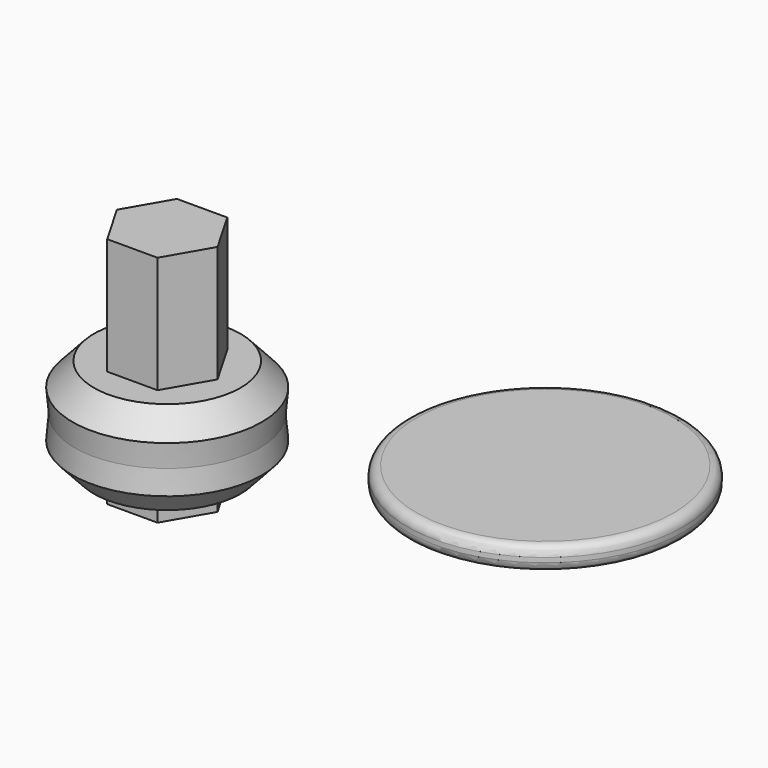
from build123d import *

# Parameters (mm, degrees)
F0_R     = 50.3856473316
F1_DEPTH = 25.4
F1_TAPER = -5
F0_R_2   = 75.1170486434
F2_DEPTH = 6.35
F4_DEPTH = 63.5
F6_R     = 5.08


# Not quite as in the source:
# - a fillet or chamfer that OpenCascade refuses, or shapes differently, is made with other operations: its cross-section is extruded or revolved along the edge and cut away or added


with BuildPart() as f1:
    # F0 (on Top) → F1 (new body, symmetric)
    with BuildSketch(Plane.XY):
        Circle(F0_R)
    extrude(amount=F1_DEPTH, both=True, taper=F1_TAPER)

    # F3 (on face) → F4 (join, symmetric)
    with BuildSketch(Plane.XY.offset(25.4)):
        Polygon((-13.6938337482, 23.7386310616), (-27.4051744245, 0.0101076296), (-13.7113406763, -23.728523432), (13.6938337482, -23.7386310616), (27.4051744245, -0.0101076296), (13.7113406763, 23.728523432), align=None)
    extrude(amount=F4_DEPTH, both=True)

    # F5: chamfer of 12.7 on 2 edges, made by hand

    # F5_s1 → F5_t2 (revolve, cut)
    with BuildSketch(Plane.XZ):
        Polygon((51.5009814523, -12.7483273342), (39.9078593852, -25.4), (52.6078593852, -25.4), align=None)
    revolve(axis=Axis((0, 0, -25.4), (0, 0, 1)), mode=Mode.SUBTRACT)

    # F5_s3 → F5_t4 (revolve, cut)
    with BuildSketch(Plane.XZ):
        Polygon((51.5009814523, 12.7483273342), (39.9078593852, 25.4), (52.6078593852, 25.4), align=None)
    revolve(axis=Axis((0, 0, 25.4), (0, 0, -1)), mode=Mode.SUBTRACT)


with BuildPart() as f2:
    # F0 (on Top) → F2 (new body, symmetric)
    with BuildSketch(Plane.XY):
        with Locations((162.7428382635, 53.8556501269)):
            Circle(F0_R_2)
    extrude(amount=F2_DEPTH, both=True)

    # F6
    f6_edges = [f2.edges().sort_by_distance(p)[0] for p in [
        (87.62579, 53.85565, -6.35),
        (87.62579, 53.85565, 6.35),
    ]]
    fillet(f6_edges, radius=F6_R)


solid = Compound([f1.part, f2.part])
